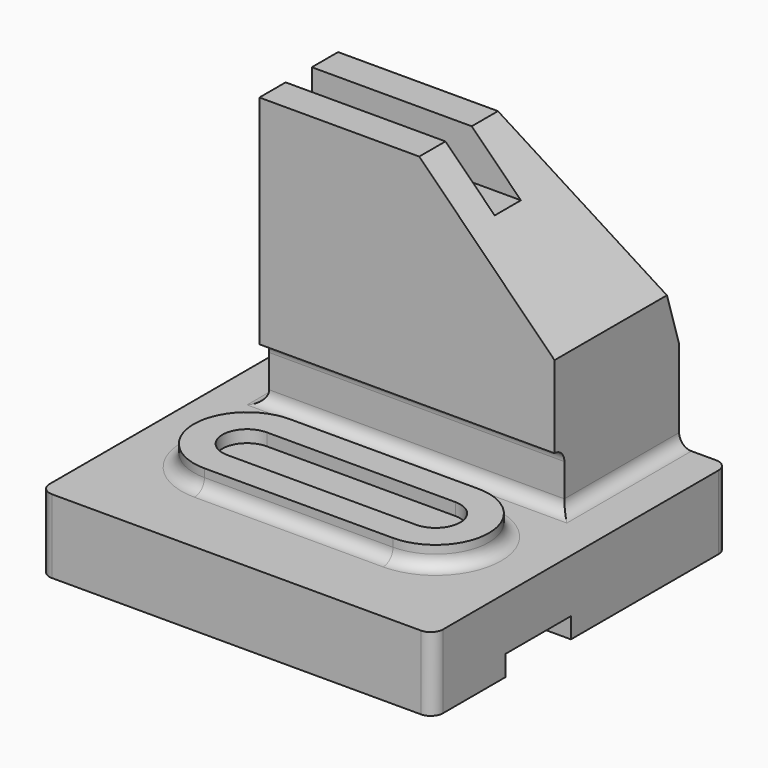
from build123d import *

# Parameters (mm, degrees)
F0_W      = 96
F0_H      = 90
F1_DEPTH  = 18
F2_W      = 72
F2_H      = 38
F4_DEPTH  = 67
F6_DEPTH  = 38
F7_W      = 8
F7_H      = 12
F8_DEPTH  = 51.001
F10_DEPTH = 72.001
F11_W     = 20
F11_H     = 5
F12_DEPTH = 96
F14_W     = 46
F14_H     = 26
F15_DEPTH = 5
F17_DEPTH = 3
F18_W     = 3
F18_H     = 14
F19_DEPTH = 72
F20_R     = 2.99999


# Not quite as in the source:
# - a fillet or chamfer is up to 0.001 mm smaller than in the source, because OpenCascade refuses the exact size


with BuildPart() as f1:
    # F0 (on Top) → F1 (new body)
    with BuildSketch(Plane.XY):
        with Locations((48, 45)):
            Rectangle(F0_W, F0_H)
    extrude(amount=F1_DEPTH)

    # F2 (on face) → F4 (join, through all)
    with BuildSketch(Plane.XY.offset(18)):
        with Locations((48, 71)):
            Rectangle(F2_W, F2_H)
    extrude(amount=F4_DEPTH)

    # F5 (on face) → F6 (cut)
    with BuildSketch(Plane.XZ.offset(-52)):
        Polygon((84, 52), (84, 85), (51, 85), align=None)
    extrude(amount=-F6_DEPTH, mode=Mode.SUBTRACT)

    # F7 (on face) → F8 (cut, through all)
    with BuildSketch(Plane(origin=(12, 0, 0), x_dir=(0, -1, 0), z_dir=(-1, 0, 0))):
        with Locations((-64, 79)):
            Rectangle(F7_W, F7_H)
    extrude(amount=-F8_DEPTH, mode=Mode.SUBTRACT)

    # F9 (on face) → F10 (cut, through all)
    with BuildSketch(Plane(origin=(12, 0, 0), x_dir=(0, -1, 0), z_dir=(-1, 0, 0))):
        Polygon((-76, 85), (-90, 85), (-90, 40), align=None)
    extrude(amount=-F10_DEPTH, mode=Mode.SUBTRACT)

    # F11 (on face) → F12 (cut, through all)
    with BuildSketch(Plane.YZ.offset(96)):
        with Locations((32, 2.5)):
            Rectangle(F11_W, F11_H)
    extrude(amount=-F12_DEPTH, mode=Mode.SUBTRACT)

    # F14 (on face) → F15 (join)
    with BuildSketch(Plane.XY.offset(18)):
        with Locations((48, 32)):
            Rectangle(F14_W, F14_H)
        with BuildLine():
            Line((25, 19), (25, 45))
            ThreePointArc((25, 45), (12, 32), (25, 19))
        make_face()
        with BuildLine():
            ThreePointArc((71, 19), (84, 32), (71, 45))
            Line((71, 45), (71, 19))
        make_face()
    extrude(amount=F15_DEPTH)

    # F16 (on face) → F17 (cut)
    with BuildSketch(Plane.XY.offset(23)):
        with BuildLine():
            ThreePointArc((25, 38), (19, 32), (25, 26))
            Line((25, 26), (71, 26))
            ThreePointArc((71, 26), (77, 32), (71, 38))
            Line((71, 38), (25, 38))
        make_face()
    extrude(amount=-F17_DEPTH, mode=Mode.SUBTRACT)

    # F18 (on face) → F19 (cut, through all)
    with BuildSketch(Plane.YZ.offset(84)):
        with Locations((53.5, 25)):
            Rectangle(F18_W, F18_H)
    extrude(amount=-F19_DEPTH, mode=Mode.SUBTRACT)

    # F20 (radius 3 in the source; OpenCascade refuses exactly that, so slightly less here)
    f20_edges = [f1.edges().sort_by_distance(p)[0] for p in [
        (48, 19, 18),
        (48, 55, 18),
        (48, 55, 32),
        (0, 0, 9),
        (96, 0, 9),
        (96, 90, 9),
        (0, 90, 9),
        (84, 72.5, 18),
        (12, 72.5, 18),
    ]]
    fillet(f20_edges, radius=F20_R)


solid = f1.part
